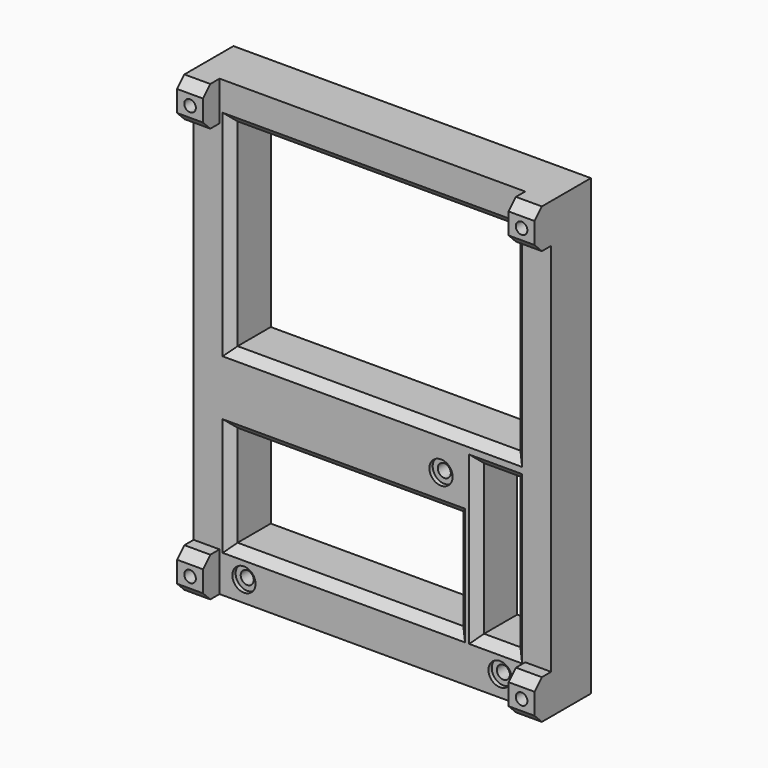
from build123d import *

# Parameters (mm, degrees)
F0_R     = 2.8
F1_DEPTH = 12
F0_W     = 6.25
F0_H     = 9.5
F0_R_2   = 1.4
F2_DEPTH = 17
F3_SIZE  = 2.2
F4_START = 8
F0_R_3   = 1.575
F4_DEPTH = 3
F5_W     = 68.25
F5_H     = 47.75
F5_W_2   = 8.775
F5_H_2   = 36.234842279
F5_W_3   = 54.475
F5_H_3   = 24.4
F6_DEPTH = 28
F7_SIZE  = 2


# Not quite as in the source:
# - a feature names something its author has since deleted; it is built from what else it names


with BuildPart() as f1:
    # F0 (on Front) → F1 (new body)
    with BuildSketch(Plane.XZ):
        Polygon((-36.875, -54.75), (36.875, -54.75), (36.875, -45.25), (43.125, -45.25), (43.125, 45.25), (36.875, 45.25), (36.875, 54.75), (-36.875, 54.75), (-36.875, 45.25), (-43.125, 45.25), (-43.125, -45.25), (-36.875, -45.25), align=None)
        with Locations((-31, -49.75)):
            Circle(F0_R, mode=Mode.SUBTRACT)
        with Locations((30.8, -49.75)):
            Circle(F0_R, mode=Mode.SUBTRACT)
        with Locations((16.55, -11.55)):
            Circle(F0_R, mode=Mode.SUBTRACT)
    extrude(amount=F1_DEPTH)

    # F0 (on Front) → F2 (join)
    with BuildSketch(Plane.XZ):
        with Locations((40, -50)):
            Rectangle(F0_W, F0_H)
        Polygon((40, -46.4492958445), (43.075, -48.2246479222), (43.075, -51.7753520778), (40, -53.5507041555), (36.925, -51.7753520778), (36.925, -48.2246479222), align=None, mode=Mode.SUBTRACT)
        with Locations((-40, -50)):
            Rectangle(F0_W, F0_H)
        Polygon((-40, -46.4492958445), (-36.925, -48.2246479222), (-36.925, -51.7753520778), (-40, -53.5507041555), (-43.075, -51.7753520778), (-43.075, -48.2246479222), align=None, mode=Mode.SUBTRACT)
        with Locations((-40, 50)):
            Rectangle(F0_W, F0_H)
        Polygon((-40, 53.5507041555), (-36.925, 51.7753520778), (-36.925, 48.2246479222), (-40, 46.4492958445), (-43.075, 48.2246479222), (-43.075, 51.7753520778), align=None, mode=Mode.SUBTRACT)
        with Locations((40, 50)):
            Rectangle(F0_W, F0_H)
        Polygon((40, 46.4492958445), (36.925, 48.2246479222), (36.925, 51.7753520778), (40, 53.5507041555), (43.075, 51.7753520778), (43.075, 48.2246479222), align=None, mode=Mode.SUBTRACT)
        Polygon((-36.925, -51.7753520778), (-36.925, -48.2246479222), (-40, -46.4492958445), (-43.075, -48.2246479222), (-43.075, -51.7753520778), (-40, -53.5507041555), align=None)
        with Locations((-40, -50)):
            Circle(F0_R_2, mode=Mode.SUBTRACT)
        Polygon((43.075, -51.7753520778), (43.075, -48.2246479222), (40, -46.4492958445), (36.925, -48.2246479222), (36.925, -51.7753520778), (40, -53.5507041555), align=None)
        with Locations((40, -50)):
            Circle(F0_R_2, mode=Mode.SUBTRACT)
        Polygon((36.925, 51.7753520778), (36.925, 48.2246479222), (40, 46.4492958445), (43.075, 48.2246479222), (43.075, 51.7753520778), (40, 53.5507041555), align=None)
        with Locations((40, 50)):
            Circle(F0_R_2, mode=Mode.SUBTRACT)
        Polygon((-36.925, 48.2246479222), (-36.925, 51.7753520778), (-40, 53.5507041555), (-43.075, 51.7753520778), (-43.075, 48.2246479222), (-40, 46.4492958445), align=None)
        with Locations((-40, 50)):
            Circle(F0_R_2, mode=Mode.SUBTRACT)
    extrude(amount=F2_DEPTH)

    # F3
    f3_edges = [f1.edges().sort_by_distance(p)[0] for p in [
        (-40, -17, -45.25),
        (-40, -17, -54.75),
        (40, -17, -45.25),
        (40, -17, -54.75),
        (-40, -17, 54.75),
        (-40, -17, 45.25),
        (40, -17, 54.75),
        (40, -17, 45.25),
    ]]
    chamfer(f3_edges, length=F3_SIZE)

    # F0 (on Front) → F4 (join)
    with BuildSketch(Plane.XZ.offset(F4_START)):
        with Locations((16.55, -11.55)):
            Circle(F0_R)
        with Locations((16.55, -11.55)):
            Circle(F0_R_3, mode=Mode.SUBTRACT)
        with Locations((30.8, -49.75)):
            Circle(F0_R)
        with Locations((30.8, -49.75)):
            Circle(F0_R_3, mode=Mode.SUBTRACT)
        with Locations((-31, -49.75)):
            Circle(F0_R)
        with Locations((-31, -49.75)):
            Circle(F0_R_3, mode=Mode.SUBTRACT)
    extrude(amount=F4_DEPTH)

    # F5 (on face) → F6 (cut)
    with BuildSketch(Plane(origin=(0, 0, 0), x_dir=(-1, 0, 0), z_dir=(0, 1, 0))):
        with Locations((0, 21.875)):
            Rectangle(F5_W, F5_H)
        with Locations((-29.7375, -25.6325788605)):
            Rectangle(F5_W_2, F5_H_2)
        with Locations((6.8875, -31.55)):
            Rectangle(F5_W_3, F5_H_3)
    extrude(amount=-F6_DEPTH, mode=Mode.SUBTRACT)

    # F7
    f7_edges = [f1.edges().sort_by_distance(p)[0] for p in [
        (0, -12, -2),
        (-34.125, -12, 21.875),
        (0, -12, 45.75),
        (34.125, -12, 21.875),
        (34.125, -12, -25.632579),
        (29.7375, -12, -7.515158),
        (25.35, -12, -25.632579),
        (29.7375, -12, -43.75),
        (-6.8875, -12, -43.75),
        (20.35, -12, -31.55),
        (-6.8875, -12, -19.35),
        (-34.125, -12, -31.55),
    ]]
    chamfer(f7_edges, length=F7_SIZE)


solid = f1.part
